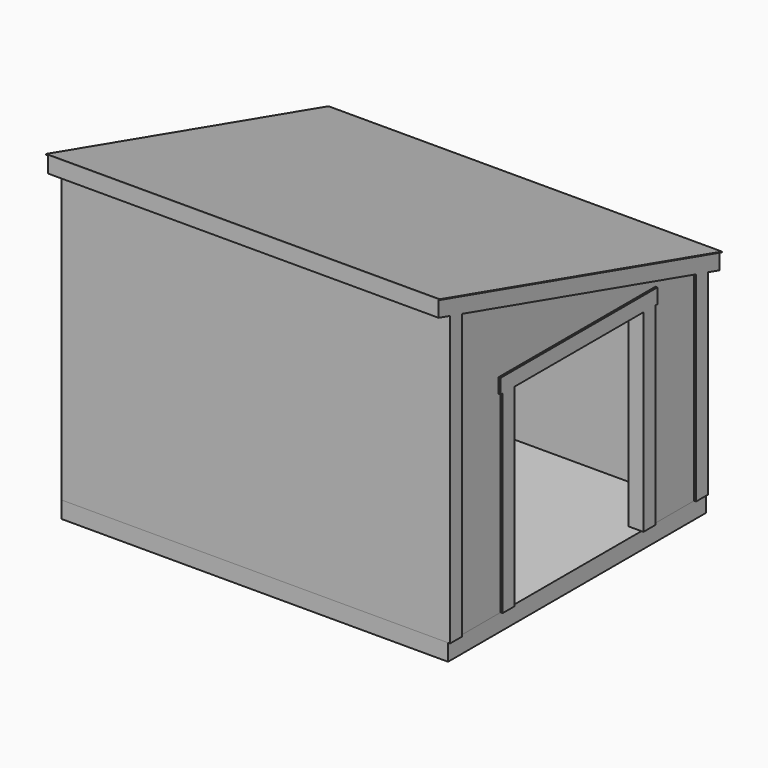
from build123d import *

# Parameters (mm, degrees)
F0_W      = 3657.6
F0_H      = 3048
F1_DEPTH  = 2880.36
F2_SIZE2  = 3047.99999
F2_SIZE   = 876.29999
F3_W      = 3695.7
F3_H      = 3454.4
F3_W_2    = 3657.6
F3_H_2    = 3171.4674224267
F6_W      = 3721.1
F6_H      = 3472.18
F7_DEPTH  = 6.35
F8_W      = 139.7
F8_H      = 1828.8
F9_DEPTH  = 19.05
F10_DEPTH = 121.92
F12_DEPTH = 3352.8
F13_W     = 3657.6
F13_H     = 3048
F14_DEPTH = 158.496


# Not quite as in the source:
# - a fillet or chamfer is up to 0.001 mm smaller than in the source, because OpenCascade refuses the exact size


with BuildPart() as f1:
    # F0 (on Top) → F1 (new body)
    with BuildSketch(Plane.XY):
        with Locations((-1828.8, 1524)):
            Rectangle(F0_W, F0_H)
    extrude(amount=F1_DEPTH)

    # F2 (size 876.3 and 3048 in the source; OpenCascade refuses exactly that, so slightly less here)
    f2_edges = [f1.edges().sort_by_distance(p)[0] for p in [
        (-1828.8, 3048, 2880.36),
    ]]
    f2_side = f1.faces().sort_by_distance((-1828.8, 3048, 1440.18))[0]
    chamfer(f2_edges, length=F2_SIZE, length2=F2_SIZE2, reference=f2_side)

    # F5: sweep along a path in F4
    with BuildLine(Plane.YZ) as f5_path:
        Line((0, 2880.36), (0, 2727.96))
    # F3 (on face) → F5 (sweep)
    with BuildSketch(Plane(origin=(0, 764.8812815702, 2660.4566315486), x_dir=(1, 0, 0), z_dir=(0, 0.2763074249, 0.9610693039))):
        with Locations((-1828.8, 789.8688630733)):
            Rectangle(F3_W, F3_H)
        with Locations((-1828.8, 789.8688664972)):
            Rectangle(F3_W_2, F3_H_2, mode=Mode.SUBTRACT)
    sweep(path=f5_path.line)

    # F6 (on face) → F7 (join)
    with BuildSketch(Plane(origin=(0, 764.8812815702, 2660.4566315486), x_dir=(1, 0, 0), z_dir=(0, 0.2763074249, 0.9610693039))):
        with Locations((-1828.8, 793.6788630733)):
            Rectangle(F6_W, F6_H)
    extrude(amount=F7_DEPTH)

    # F8 (on face) → F9 (join)
    with BuildSketch(Plane.YZ):
        Polygon((0, 2727.96), (0, 0), (139.7, 0), (139.7, 2687.79625), align=None)
        Polygon((2908.3, 0), (3048, 0), (3048, 1851.66), (2908.3, 1891.82375), align=None)
        with Locations((692.15, 914.4)):
            Rectangle(F8_W, F8_H)
        Polygon((622.3, 1828.8), (762, 1828.8), (1524, 1828.8), (2286, 1828.8), (2425.7, 1828.8), (2451.1, 1828.8), (2451.1, 1968.5), (1524, 1968.5), (596.9, 1968.5), (596.9, 1828.8), align=None)
        with Locations((2355.85, 914.4)):
            Rectangle(F8_W, F8_H)
    extrude(amount=F9_DEPTH)

    # F10 (cut): a face of the model
    f10_faces = [f1.faces().sort_by_distance(p)[0] for p in [
        (0, 1524, 914.4),
    ]]
    extrude(f10_faces, amount=-F10_DEPTH, mode=Mode.SUBTRACT)

    # F11 (on face) → F12 (cut)
    with BuildSketch(Plane.YZ.offset(-121.92)):
        Polygon((198.8992989063, 0), (2843.3250255278, 0), (2843.3250255278, 2012.4011538445), (198.8992989063, 2772.6735502481), align=None)
    extrude(amount=-F12_DEPTH, mode=Mode.SUBTRACT)


with BuildPart() as f14:
    # F13 (on Top) → F14 (new body)
    with BuildSketch(Plane.XY):
        with Locations((-1828.8, 1524)):
            Rectangle(F13_W, F13_H)
    extrude(amount=-F14_DEPTH)


solid = Compound([f1.part, f14.part])
